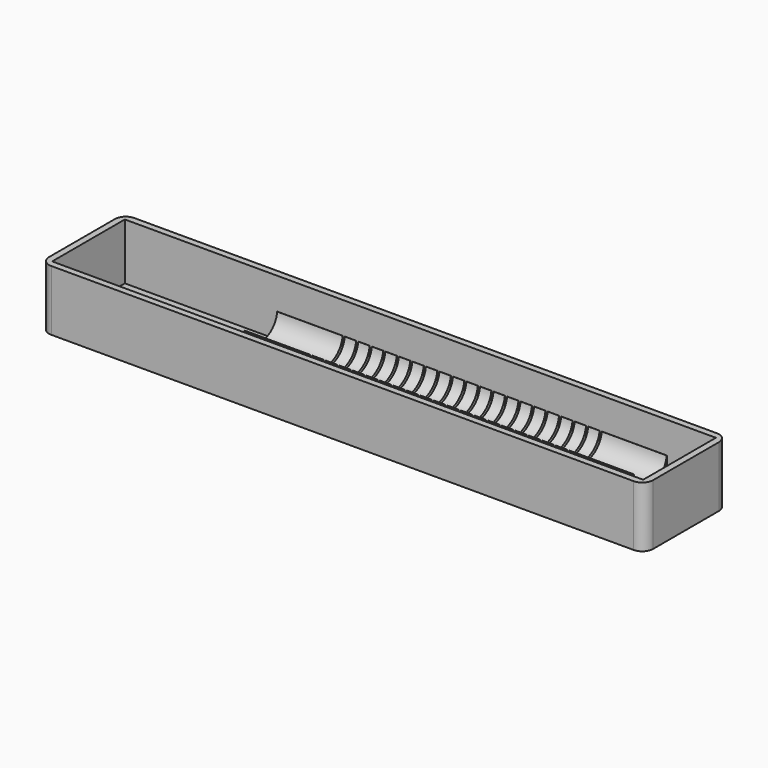
from build123d import *

# Parameters (mm, degrees)
F0_W      = 30.2304342687
F0_H      = 19
F0_W_2    = 0.5
F0_W_3    = 5.25
F0_W_4    = 30.0195657313
F1_DEPTH  = 15
F0_W_5    = 6.6043436527
F0_H_2    = 2.9876781628
F0_W_6    = 51
F0_H_3    = 18
F0_W_7    = 6.3103074431
F3_DEPTH  = 2
F4_R      = 9.5
F5_DEPTH  = 180
F2_W      = 0.5
F2_H      = 19
F7_DEPTH  = 10
F6_W      = 8.3426982164
F6_H      = 1.8960679881
F8_DEPTH  = 19
F0_W_8    = 279.1266992456
F0_H_4    = 48
F9_DEPTH  = 28
F10_W     = 1.7696609721
F10_H     = 6.1938203871
F11_DEPTH = 5
F12_R     = 5


# Not quite as in the source:
# - a feature names something its author has since deleted; it is built from what else it names


with BuildPart() as f1:
    # F0 (on Top) → F1 (new body)
    with BuildSketch(Plane.XY):
        with Locations((-58.5658399016, 6.1430045813)):
            Rectangle(F0_W, F0_H)
        with Locations((-43.2006227672, 6.1430045813)):
            Rectangle(F0_W_2, F0_H)
        with Locations((-42.7006227672, 6.1430045813)):
            Rectangle(F0_W_2, F0_H)
        with Locations((-39.8256227672, 6.1430045813)):
            Rectangle(F0_W_3, F0_H)
        with Locations((-36.9506227672, 6.1430045813)):
            Rectangle(F0_W_2, F0_H)
        with Locations((-36.4506227672, 6.1430045813)):
            Rectangle(F0_W_2, F0_H)
        with Locations((-33.5756227672, 6.1430045813)):
            Rectangle(F0_W_3, F0_H)
        with Locations((-30.7006227672, 6.1430045813)):
            Rectangle(F0_W_2, F0_H)
        with Locations((-30.2006227672, 6.1430045813)):
            Rectangle(F0_W_2, F0_H)
        with Locations((-27.3256227672, 6.1430045813)):
            Rectangle(F0_W_3, F0_H)
        with Locations((-24.4506227672, 6.1430045813)):
            Rectangle(F0_W_2, F0_H)
        with Locations((-23.9506227672, 6.1430045813)):
            Rectangle(F0_W_2, F0_H)
        with Locations((-21.0756227672, 6.1430045813)):
            Rectangle(F0_W_3, F0_H)
        with Locations((-18.2006227672, 6.1430045813)):
            Rectangle(F0_W_2, F0_H)
        with Locations((-17.7006227672, 6.1430045813)):
            Rectangle(F0_W_2, F0_H)
        with Locations((-14.8256227672, 6.1430045813)):
            Rectangle(F0_W_3, F0_H)
        with Locations((-11.9506227672, 6.1430045813)):
            Rectangle(F0_W_2, F0_H)
        with Locations((-11.4506227672, 6.1430045813)):
            Rectangle(F0_W_2, F0_H)
        with Locations((-8.5756227672, 6.1430045813)):
            Rectangle(F0_W_3, F0_H)
        with Locations((-5.7006227672, 6.1430045813)):
            Rectangle(F0_W_2, F0_H)
        with Locations((-5.2006227672, 6.1430045813)):
            Rectangle(F0_W_2, F0_H)
        with Locations((-2.3256227672, 6.1430045813)):
            Rectangle(F0_W_3, F0_H)
        with Locations((0.5493772328, 6.1430045813)):
            Rectangle(F0_W_2, F0_H)
        with Locations((1.0493772328, 6.1430045813)):
            Rectangle(F0_W_2, F0_H)
        with Locations((3.9243772328, 6.1430045813)):
            Rectangle(F0_W_3, F0_H)
        with Locations((6.7993772328, 6.1430045813)):
            Rectangle(F0_W_2, F0_H)
        with Locations((7.2993772328, 6.1430045813)):
            Rectangle(F0_W_2, F0_H)
        with Locations((10.1743772328, 6.1430045813)):
            Rectangle(F0_W_3, F0_H)
        with Locations((13.0493772328, 6.1430045813)):
            Rectangle(F0_W_2, F0_H)
        with Locations((13.5493772328, 6.1430045813)):
            Rectangle(F0_W_2, F0_H)
        with Locations((16.4243772328, 6.1430045813)):
            Rectangle(F0_W_3, F0_H)
        with Locations((19.2993772328, 6.1430045813)):
            Rectangle(F0_W_2, F0_H)
        with Locations((19.7993772328, 6.1430045813)):
            Rectangle(F0_W_2, F0_H)
        with Locations((22.6743772328, 6.1430045813)):
            Rectangle(F0_W_3, F0_H)
        with Locations((25.5493772328, 6.1430045813)):
            Rectangle(F0_W_2, F0_H)
        with Locations((26.0493772328, 6.1430045813)):
            Rectangle(F0_W_2, F0_H)
        with Locations((28.9243772328, 6.1430045813)):
            Rectangle(F0_W_3, F0_H)
        with Locations((31.7993772328, 6.1430045813)):
            Rectangle(F0_W_2, F0_H)
        with Locations((32.2993772328, 6.1430045813)):
            Rectangle(F0_W_2, F0_H)
        with Locations((35.1743772328, 6.1430045813)):
            Rectangle(F0_W_3, F0_H)
        with Locations((38.0493772328, 6.1430045813)):
            Rectangle(F0_W_2, F0_H)
        with Locations((38.5493772328, 6.1430045813)):
            Rectangle(F0_W_2, F0_H)
        with Locations((41.4243772328, 6.1430045813)):
            Rectangle(F0_W_3, F0_H)
        with Locations((44.2993772328, 6.1430045813)):
            Rectangle(F0_W_2, F0_H)
        with Locations((44.7993772328, 6.1430045813)):
            Rectangle(F0_W_2, F0_H)
        with Locations((47.6743772328, 6.1430045813)):
            Rectangle(F0_W_3, F0_H)
        with Locations((50.5493772328, 6.1430045813)):
            Rectangle(F0_W_2, F0_H)
        with Locations((51.0493772328, 6.1430045813)):
            Rectangle(F0_W_2, F0_H)
        with Locations((53.9243772328, 6.1430045813)):
            Rectangle(F0_W_3, F0_H)
        with Locations((56.7993772328, 6.1430045813)):
            Rectangle(F0_W_2, F0_H)
        with Locations((57.2993772328, 6.1430045813)):
            Rectangle(F0_W_2, F0_H)
        with Locations((60.1743772328, 6.1430045813)):
            Rectangle(F0_W_3, F0_H)
        with Locations((63.0493772328, 6.1430045813)):
            Rectangle(F0_W_2, F0_H)
        with Locations((63.5493772328, 6.1430045813)):
            Rectangle(F0_W_2, F0_H)
        with Locations((66.4243772328, 6.1430045813)):
            Rectangle(F0_W_3, F0_H)
        with Locations((69.2993772328, 6.1430045813)):
            Rectangle(F0_W_2, F0_H)
        with Locations((69.7993772328, 6.1430045813)):
            Rectangle(F0_W_2, F0_H)
        with Locations((72.6743772328, 6.1430045813)):
            Rectangle(F0_W_3, F0_H)
        with Locations((75.5493772328, 6.1430045813)):
            Rectangle(F0_W_2, F0_H)
        with Locations((76.0493772328, 6.1430045813)):
            Rectangle(F0_W_2, F0_H)
        with Locations((91.3091600984, 6.1430045813)):
            Rectangle(F0_W_4, F0_H)
    extrude(amount=F1_DEPTH)

    # F0 (on Top) → F3 (join)
    with BuildSketch(Plane.XY):
        Polygon((-146.0105562806, -24), (127.116142965, -24), (127.116142965, 18), (-92.0105562806, 18), (-92.0105562806, -3), (-146.0105562806, -3), (-146.0105562806, -8.9827831835), (-139.7002488375, -8.9827831835), (-139.7002488375, -11.9704613462), (-146.0105562806, -11.9704613462), align=None)
        with Locations((-95.1995551586, -10.7911149971)):
            Rectangle(F0_W_5, F0_H_2, mode=Mode.SUBTRACT)
        Polygon((-73.6810570359, -3.3569954187), (-73.6810570359, 15.6430045813), (-43.4506227672, 15.6430045813), (-42.9506227672, 15.6430045813), (-42.4506227672, 15.6430045813), (-37.2006227672, 15.6430045813), (-36.7006227672, 15.6430045813), (-36.2006227672, 15.6430045813), (-30.9506227672, 15.6430045813), (-30.4506227672, 15.6430045813), (-29.9506227672, 15.6430045813), (-24.7006227672, 15.6430045813), (-24.2006227672, 15.6430045813), (-23.7006227672, 15.6430045813), (-18.4506227672, 15.6430045813), (-17.9506227672, 15.6430045813), (-17.4506227672, 15.6430045813), (-12.2006227672, 15.6430045813), (-11.7006227672, 15.6430045813), (-11.2006227672, 15.6430045813), (-5.9506227672, 15.6430045813), (-5.4506227672, 15.6430045813), (-4.9506227672, 15.6430045813), (0.2993772328, 15.6430045813), (0.7993772328, 15.6430045813), (1.2993772328, 15.6430045813), (6.5493772328, 15.6430045813), (7.0493772328, 15.6430045813), (7.5493772328, 15.6430045813), (12.7993772328, 15.6430045813), (13.2993772328, 15.6430045813), (13.7993772328, 15.6430045813), (19.0493772328, 15.6430045813), (19.5493772328, 15.6430045813), (20.0493772328, 15.6430045813), (25.2993772328, 15.6430045813), (25.7993772328, 15.6430045813), (26.2993772328, 15.6430045813), (31.5493772328, 15.6430045813), (32.0493772328, 15.6430045813), (32.5493772328, 15.6430045813), (37.7993772328, 15.6430045813), (38.2993772328, 15.6430045813), (38.7993772328, 15.6430045813), (44.0493772328, 15.6430045813), (44.5493772328, 15.6430045813), (45.0493772328, 15.6430045813), (50.2993772328, 15.6430045813), (50.7993772328, 15.6430045813), (51.2993772328, 15.6430045813), (56.5493772328, 15.6430045813), (57.0493772328, 15.6430045813), (57.5493772328, 15.6430045813), (62.7993772328, 15.6430045813), (63.2993772328, 15.6430045813), (63.7993772328, 15.6430045813), (69.0493772328, 15.6430045813), (69.5493772328, 15.6430045813), (70.0493772328, 15.6430045813), (75.2993772328, 15.6430045813), (75.7993772328, 15.6430045813), (76.2993772328, 15.6430045813), (106.3189429641, 15.6430045813), (106.3189429641, -3.3569954187), (76.2993772328, -3.3569954187), (75.7993772328, -3.3569954187), (75.2993772328, -3.3569954187), (70.0493772328, -3.3569954187), (69.5493772328, -3.3569954187), (69.0493772328, -3.3569954187), (63.7993772328, -3.3569954187), (63.2993772328, -3.3569954187), (62.7993772328, -3.3569954187), (57.5493772328, -3.3569954187), (57.0493772328, -3.3569954187), (56.5493772328, -3.3569954187), (51.2993772328, -3.3569954187), (50.7993772328, -3.3569954187), (50.2993772328, -3.3569954187), (45.0493772328, -3.3569954187), (44.5493772328, -3.3569954187), (44.0493772328, -3.3569954187), (38.7993772328, -3.3569954187), (38.2993772328, -3.3569954187), (37.7993772328, -3.3569954187), (32.5493772328, -3.3569954187), (32.0493772328, -3.3569954187), (31.5493772328, -3.3569954187), (26.2993772328, -3.3569954187), (25.7993772328, -3.3569954187), (25.2993772328, -3.3569954187), (20.0493772328, -3.3569954187), (19.5493772328, -3.3569954187), (19.0493772328, -3.3569954187), (13.7993772328, -3.3569954187), (13.2993772328, -3.3569954187), (12.7993772328, -3.3569954187), (7.5493772328, -3.3569954187), (7.0493772328, -3.3569954187), (6.5493772328, -3.3569954187), (1.2993772328, -3.3569954187), (0.7993772328, -3.3569954187), (0.2993772328, -3.3569954187), (-4.9506227672, -3.3569954187), (-5.4506227672, -3.3569954187), (-5.9506227672, -3.3569954187), (-11.2006227672, -3.3569954187), (-11.7006227672, -3.3569954187), (-12.2006227672, -3.3569954187), (-17.4506227672, -3.3569954187), (-17.9506227672, -3.3569954187), (-18.4506227672, -3.3569954187), (-23.7006227672, -3.3569954187), (-24.2006227672, -3.3569954187), (-24.7006227672, -3.3569954187), (-29.9506227672, -3.3569954187), (-30.4506227672, -3.3569954187), (-30.9506227672, -3.3569954187), (-36.2006227672, -3.3569954187), (-36.7006227672, -3.3569954187), (-37.2006227672, -3.3569954187), (-42.4506227672, -3.3569954187), (-42.9506227672, -3.3569954187), (-43.4506227672, -3.3569954187), align=None, mode=Mode.SUBTRACT)
        with Locations((-120.5105562806, 9)):
            Rectangle(F0_W_6, F0_H_3)
        Polygon((-92.0105562806, -3), (-92.0105562806, 18), (-95.0105562806, 18), (-95.0105562806, 0), (-146.0105562806, 0), (-146.0105562806, -3), align=None)
        with Locations((-142.855402559, -10.4766222648)):
            Rectangle(F0_W_7, F0_H_2)
        with Locations((-95.1995551586, -10.7911149971)):
            Rectangle(F0_W_5, F0_H_2)
    extrude(amount=F3_DEPTH)

    # F4 (on face) → F5 (cut)
    with BuildSketch(Plane(origin=(-73.6810570359, 0, 0), x_dir=(0, -1, 0), z_dir=(-1, 0, 0))):
        with Locations((-6.1430045813, 16)):
            Circle(F4_R)
    extrude(amount=-F5_DEPTH, mode=Mode.SUBTRACT)

    # F2 (on face) → F7 (cut)
    with BuildSketch(Plane.XY.offset(15)):
        with Locations((-43.2006190121, 6.1430045813)):
            Rectangle(F2_W, F2_H)
        with Locations((-42.7006190121, 6.1430045813)):
            Rectangle(F2_W, F2_H)
        with Locations((-36.9506190121, 6.1430045813)):
            Rectangle(F2_W, F2_H)
        with Locations((-36.4506190121, 6.1430045813)):
            Rectangle(F2_W, F2_H)
        with Locations((-30.7006190121, 6.1430045813)):
            Rectangle(F2_W, F2_H)
        with Locations((-30.2006190121, 6.1430045813)):
            Rectangle(F2_W, F2_H)
        with Locations((-24.4506190121, 6.1430045813)):
            Rectangle(F2_W, F2_H)
        with Locations((-23.9506190121, 6.1430045813)):
            Rectangle(F2_W, F2_H)
        with Locations((-18.2006190121, 6.1430045813)):
            Rectangle(F2_W, F2_H)
        with Locations((-17.7006190121, 6.1430045813)):
            Rectangle(F2_W, F2_H)
        with Locations((-11.9506190121, 6.1430045813)):
            Rectangle(F2_W, F2_H)
        with Locations((-11.4506190121, 6.1430045813)):
            Rectangle(F2_W, F2_H)
        with Locations((-5.7006190121, 6.1430045813)):
            Rectangle(F2_W, F2_H)
        with Locations((-5.2006190121, 6.1430045813)):
            Rectangle(F2_W, F2_H)
        with Locations((0.5493809879, 6.1430045813)):
            Rectangle(F2_W, F2_H)
        with Locations((1.0493809879, 6.1430045813)):
            Rectangle(F2_W, F2_H)
        with Locations((6.7993809879, 6.1430045813)):
            Rectangle(F2_W, F2_H)
        with Locations((7.2993809879, 6.1430045813)):
            Rectangle(F2_W, F2_H)
        with Locations((13.0493809879, 6.1430045813)):
            Rectangle(F2_W, F2_H)
        with Locations((13.5493809879, 6.1430045813)):
            Rectangle(F2_W, F2_H)
        with Locations((19.2993809879, 6.1430045813)):
            Rectangle(F2_W, F2_H)
        with Locations((19.7993809879, 6.1430045813)):
            Rectangle(F2_W, F2_H)
        with Locations((25.5493809879, 6.1430045813)):
            Rectangle(F2_W, F2_H)
        with Locations((26.0493809879, 6.1430045813)):
            Rectangle(F2_W, F2_H)
        with Locations((31.7993809879, 6.1430045813)):
            Rectangle(F2_W, F2_H)
        with Locations((32.2993809879, 6.1430045813)):
            Rectangle(F2_W, F2_H)
        with Locations((38.0493809879, 6.1430045813)):
            Rectangle(F2_W, F2_H)
        with Locations((38.5493809879, 6.1430045813)):
            Rectangle(F2_W, F2_H)
        with Locations((44.2993809879, 6.1430045813)):
            Rectangle(F2_W, F2_H)
        with Locations((44.7993809879, 6.1430045813)):
            Rectangle(F2_W, F2_H)
        with Locations((50.5493809879, 6.1430045813)):
            Rectangle(F2_W, F2_H)
        with Locations((51.0493809879, 6.1430045813)):
            Rectangle(F2_W, F2_H)
        with Locations((56.7993809879, 6.1430045813)):
            Rectangle(F2_W, F2_H)
        with Locations((57.2993809879, 6.1430045813)):
            Rectangle(F2_W, F2_H)
        with Locations((63.0493809879, 6.1430045813)):
            Rectangle(F2_W, F2_H)
        with Locations((63.5493809879, 6.1430045813)):
            Rectangle(F2_W, F2_H)
        with Locations((69.2993809879, 6.1430045813)):
            Rectangle(F2_W, F2_H)
        with Locations((69.7993809879, 6.1430045813)):
            Rectangle(F2_W, F2_H)
        with Locations((75.5493809879, 6.1430045813)):
            Rectangle(F2_W, F2_H)
        with Locations((76.0493809879, 6.1430045813)):
            Rectangle(F2_W, F2_H)
    extrude(amount=-F7_DEPTH, mode=Mode.SUBTRACT)

    # F6 (on face) → F8 (cut)
    with BuildSketch(Plane(origin=(0, 15.6430045813, 0), x_dir=(-1, 0, 0), z_dir=(0, 1, 0))):
        with Locations((-59.220507741, 4.6769666951)):
            Rectangle(F6_W, F6_H)
        with Locations((59.220507741, 4.6769666951)):
            Rectangle(F6_W, F6_H)
    extrude(amount=-F8_DEPTH, mode=Mode.SUBTRACT)

    # F0 (on Top) → F9 (join)
    with BuildSketch(Plane.XY):
        with Locations((-9.4472066578, -3)):
            Rectangle(F0_W_8, F0_H_4)
        Polygon((127.116142965, 18), (127.116142965, -24), (-146.0105562806, -24), (-146.0105562806, -11.9704613462), (-146.0105562806, -8.9827831835), (-146.0105562806, -3), (-146.0105562806, 0), (-146.0105562806, 18), (-95.0105562806, 18), (-92.0105562806, 18), align=None, mode=Mode.SUBTRACT)
    extrude(amount=F9_DEPTH)

    # F10 (on face) → F11 (cut, symmetric)
    with BuildSketch(Plane(origin=(-149.0105562806, 0, 0), x_dir=(0, -1, 0), z_dir=(-1, 0, 0))):
        with Locations((4.2005600408, 6.9522475824)):
            Rectangle(F10_W, F10_H)
    extrude(amount=F11_DEPTH, both=True, mode=Mode.SUBTRACT)

    # F12
    f12_edges = [f1.edges().sort_by_distance(p)[0] for p in [
        (-149.010556, 21, 14),
        (130.116143, 21, 14),
        (-149.010556, -27, 14),
        (130.116143, -27, 14),
    ]]
    fillet(f12_edges, radius=F12_R)


solid = f1.part
